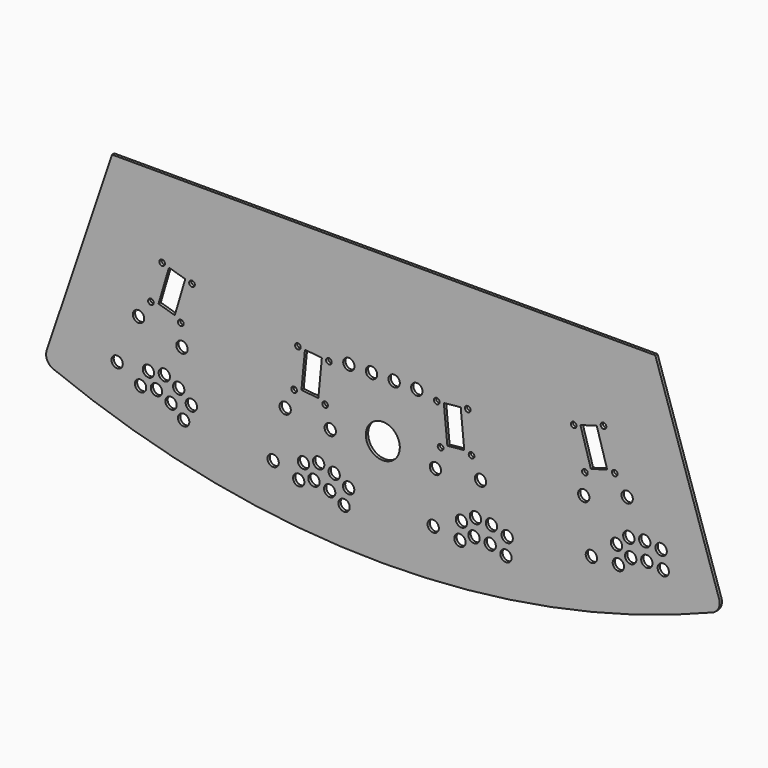
from build123d import *

# Parameters (mm, degrees)
F1_DEPTH        = 6.35
F2_R            = 12.7
F2_R_2          = 6.35
F3_DEPTH        = 6.351
F3_COPIES_COUNT = 4
F3_COPIES_ANGLE = 33
F6_R            = 38.1
F6_R_2          = 12.7
F7_DEPTH        = 6.351


# Not quite as in the source:
# - a pattern or mirror of a feature is missing from the dataset's text; its kind, count and spacing are read off the source's solid


with BuildPart() as f1:
    # F0 (on Front) → F1 (new body)
    with BuildSketch(Plane.XZ):
        with BuildLine():
            Line((611.4011750653, 0), (-607.7988249347, 0))
            Line((-607.7988249347, 0), (-754.3820135261, -434.6129904367))
            ThreePointArc((-754.3820135261, -434.6129904367), (-753.3868164341, -453.3515552834), (-739.7986522476, -466.2931944302))
            ThreePointArc((-739.7986522476, -466.2931944302), (0.0854683246, -609.5999981565), (739.9572217249, -466.2293582423))
            ThreePointArc((739.9572217249, -466.2293582423), (753.5060114552, -453.3692838691), (754.5955072236, -434.7208465349))
            Line((754.5955072236, -434.7208465349), (611.4011750653, 0))
        make_face()
    extrude(amount=F1_DEPTH)

    # F2 (on face) → F3 (cut, through all)
    with BuildSketch(Plane.XZ.offset(6.35)):
        with Locations((624.5911696341, -379.2573002913)):
            Circle(F2_R)
        with Locations((629.293420012, -418.017962579)):
            Circle(F2_R)
        with Locations((587.7311349843, -374.5315110857)):
            Circle(F2_R)
        with Locations((592.4333853621, -413.2921733735)):
            Circle(F2_R)
        with Locations((551.9889335366, -378.8611260422)):
            Circle(F2_R)
        with Locations((556.2118480679, -417.7637740763)):
            Circle(F2_R)
        with Locations((524.3242327175, -401.6570658257)):
            Circle(F2_R)
        with Locations((528.5470741868, -440.5597355017)):
            Circle(F2_R)
        with Locations((468.0006088828, -443.8931335302)):
            Circle(F2_R)
        with Locations((450.8607480357, -329.3439521574)):
            Circle(F2_R)
        with Locations((548.2768330983, -300.4879931354)):
            Circle(F2_R)
        Polygon((479.9608602999, -181.6468686851), (443.4298284015, -192.4678533183), (466.8752951068, -271.6184224317), (503.4063270052, -260.7974377985), align=None)
        with Locations((453.4575292546, -282.2156713453)):
            Circle(F2_R_2)
        with Locations((520.4310877351, -262.3771995177)):
            Circle(F2_R_2)
        with Locations((428.2085651104, -196.9765969155)):
            Circle(F2_R_2)
        with Locations((495.182123591, -177.138125088)):
            Circle(F2_R_2)
    f3 = extrude(amount=-F3_DEPTH, mode=Mode.SUBTRACT)

    # F3_copies: F3 ×4 about axis
    f3_copies_axis = Axis((0.085468, 0, 1371.6), (0, 1, 0))
    for i in range(1, F3_COPIES_COUNT):
        add(f3.rotate(f3_copies_axis, i * F3_COPIES_ANGLE / (F3_COPIES_COUNT - 1)), mode=Mode.SUBTRACT)

    # F6 (on face) → F7 (cut, through all)
    with BuildSketch(Plane.XZ.offset(6.35)):
        with Locations((0, -368.3)):
            Circle(F6_R)
        with Locations((-76.2, -241.3)):
            Circle(F6_R_2)
        with Locations((-25.4, -241.3)):
            Circle(F6_R_2)
        with Locations((25.4, -241.3)):
            Circle(F6_R_2)
        with Locations((76.2, -241.3)):
            Circle(F6_R_2)
    extrude(amount=-F7_DEPTH, mode=Mode.SUBTRACT)


solid = f1.part
